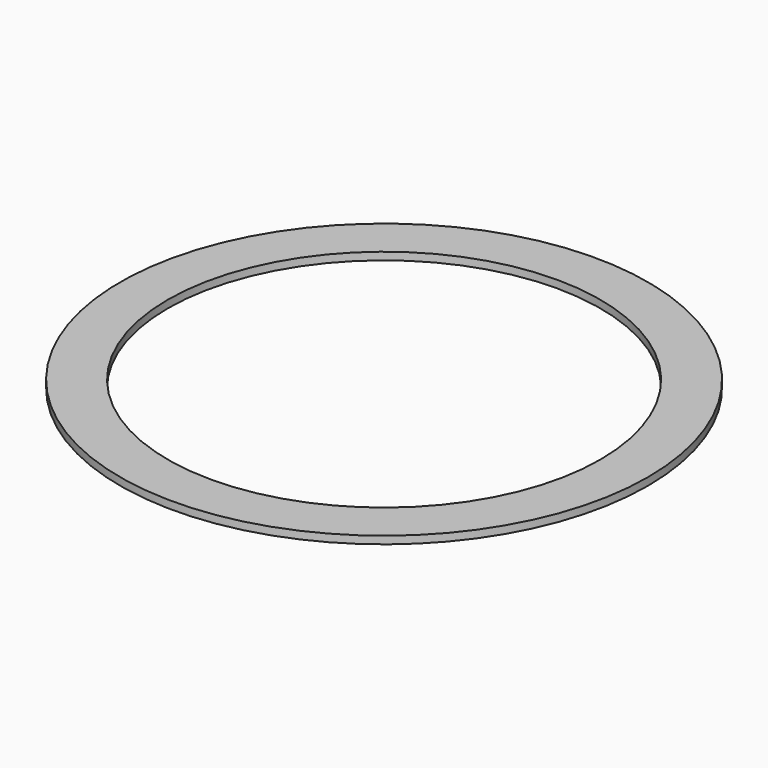
from build123d import *

# Parameters (mm, degrees)
F0_R     = 165.1
F0_R_2   = 135.32739
F1_DEPTH = 4.7625


# Not quite as in the source:
# - a length typed as a fraction of an inch, garbled in the dataset ("3 / 203.2 mm" for 3/8 in), is restored


with BuildPart() as f1:
    # F0 (on Top) → F1 (new body)
    with BuildSketch(Plane.XY):
        Circle(F0_R)
        Circle(F0_R_2, mode=Mode.SUBTRACT)
    extrude(amount=F1_DEPTH)


solid = f1.part
